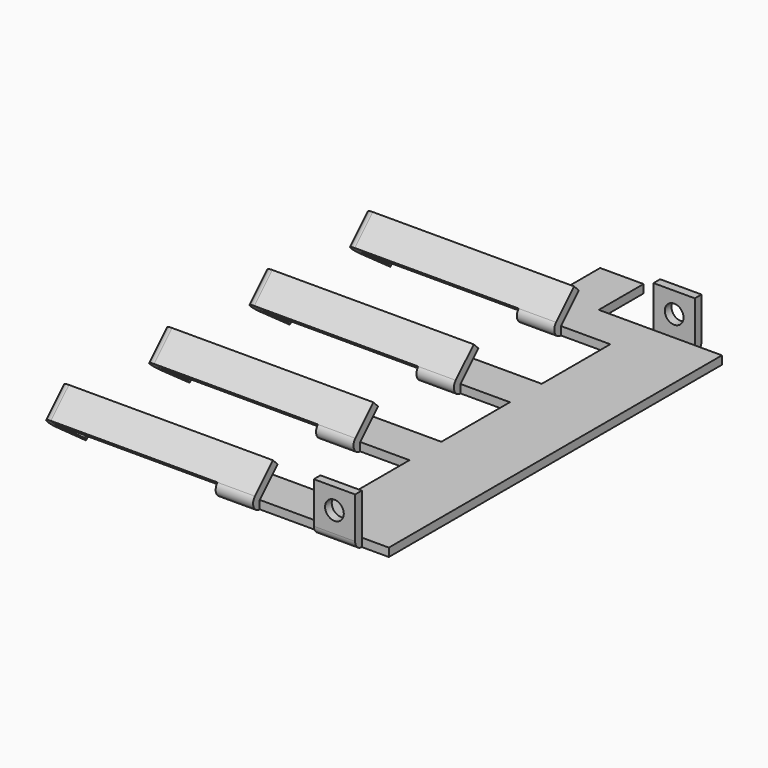
from build123d import *

# Parameters (mm, degrees)
F1_DEPTH  = 1
F3_DEPTH  = 40
F5_DEPTH  = 7.6454254
F8_DEPTH  = 8.9916
F9_DEPTH  = 39.37
F11_REACH = 42.1217729552
F13_REACH = 63.4368099505
F15_REACH = 84.7531019793
F16_W     = 9.9314
F16_H     = 11.938
F17_DEPTH = 2
F18_W     = 9.9314
F18_H     = 11.938
F19_DEPTH = 2
F20_R     = 2
F22_D     = 4.5


with BuildPart() as f1:
    # F0 (on Top) → F1 (new body, symmetric)
    with BuildSketch(Plane.XY):
        Polygon((40, -50), (40, 50), (10.4203875556, 50), (10.4203875556, 63.4358227253), (0, 63.4358227253), (0, 50), (0, 40.4320432043), (20.8407751113, 40.4320432043), (20.8407751113, 19.8559855986), (0, 19.8559855986), (0, 10.2880288029), (20.8407751113, 10.2880288029), (20.8407751113, -10.2880288029), (0, -10.2880288029), (0, -19.8559855986), (20.8407751113, -19.8559855986), (20.8407751113, -40.4320432043), (0, -40.4320432043), (0, -50), align=None)
    extrude(amount=F1_DEPTH, both=True)

    # F2 (on Right) → F3 (join)
    with BuildSketch(Plane.YZ):
        Polygon((-50, 1), (-50, 0.9964082731), (-44.6311706177, 6.3652376554), (-46.04538418, 7.7794512178), (-51.4515079706, 2.3733274272), align=None)
    extrude(amount=-F3_DEPTH)

    # F4 (on face) → F5 (join)
    with BuildSketch(Plane(origin=(0, -19.1329664811, -19.1329664811), x_dir=(1, 0, 0), z_dir=(0, 0.7071067812, 0.7071067812))):
        with BuildLine():
            Line((-34.9300994608, -32.0862576741), (-40.6840402867, -34.1805208645))
            ThreePointArc((-40.6840402867, -34.1805208645), (-41.969615506, -36.4072024614), (-40, -38.059906106))
            Line((-40, -38.059906106), (-40, -36.059906106))
            Line((-40, -36.059906106), (-34.2460591741, -33.9656429157))
            Line((-34.2460591741, -33.9656429157), (-34.9300994608, -32.0862576741))
        make_face()
    extrude(amount=-F5_DEPTH)

    # F6 (on Right) + F2 (on Right) + F7 (on Right) → F8 (join)
    with BuildSketch(Plane.YZ):
        Polygon((-19.8559855986, 0.9982251152), (-19.8559855986, 0.9946333883), (-14.4871562162, 6.3634627706), (-15.9013697786, 7.777676333), (-21.3074935692, 2.3715525424), align=None)
        with BuildLine():
            Line((-19.8559855986, -1), (-19.8559855986, 0.9946333883))
            Line((-19.8559855986, 0.9946333883), (-19.8559855986, 0.9982251152))
            Line((-19.8559855986, 0.9982251152), (-21.3074935692, 2.3715525424))
            ThreePointArc((-21.3074935692, 2.3715525424), (-21.6913494545, 0.2080712521), (-19.8559855986, -1))
        make_face()
    with BuildSketch(Plane.YZ):
        Polygon((-50, 1), (-50, 0.9964082731), (-44.6311706177, 6.3652376554), (-46.04538418, 7.7794512178), (-51.4515079706, 2.3733274272), align=None)
        with BuildLine():
            Line((-50, -0.9982251152), (-50, 0.9964082731))
            Line((-50, 0.9964082731), (-50, 1))
            Line((-50, 1), (-51.4515079706, 2.3733274272))
            ThreePointArc((-51.4515079706, 2.3733274272), (-51.8353638559, 0.2098461369), (-50, -0.9982251152))
        make_face()
    with BuildSketch(Plane.YZ):
        Polygon((10.2880288029, 0.9982251152), (10.2880288029, 0.9946333883), (15.6568581852, 6.3634627706), (14.2426446228, 7.777676333), (8.8365208322, 2.3715525424), align=None)
        with BuildLine():
            Line((10.2880288029, -1), (10.2880288029, 0.9946333883))
            Line((10.2880288029, 0.9946333883), (10.2880288029, 0.9982251152))
            Line((10.2880288029, 0.9982251152), (8.8365208322, 2.3715525424))
            ThreePointArc((8.8365208322, 2.3715525424), (8.4526649469, 0.2080712521), (10.2880288029, -1))
        make_face()
        Polygon((40.4320432043, 1), (40.4320432043, 0.9964082731), (45.8008725867, 6.3652376554), (44.3866590243, 7.7794512177), (38.9805352337, 2.3733274272), align=None)
        with BuildLine():
            Line((40.4320432043, -0.9982251152), (40.4320432043, 0.9964082731))
            Line((40.4320432043, 0.9964082731), (40.4320432043, 1))
            Line((40.4320432043, 1), (38.9805352337, 2.3733274272))
            ThreePointArc((38.9805352337, 2.3733274272), (38.5966793484, 0.2098461369), (40.4320432043, -0.9982251152))
        make_face()
    extrude(amount=F8_DEPTH)

    # F6 (on Right) + F7 (on Right) → F9 (join)
    with BuildSketch(Plane.YZ):
        Polygon((-19.8559855986, 0.9982251152), (-19.8559855986, 0.9946333883), (-14.4871562162, 6.3634627706), (-15.9013697786, 7.777676333), (-21.3074935692, 2.3715525424), align=None)
    with BuildSketch(Plane.YZ):
        Polygon((10.2880288029, 0.9982251152), (10.2880288029, 0.9946333883), (15.6568581852, 6.3634627706), (14.2426446228, 7.777676333), (8.8365208322, 2.3715525424), align=None)
        Polygon((40.4320432043, 1), (40.4320432043, 0.9964082731), (45.8008725867, 6.3652376554), (44.3866590243, 7.7794512177), (38.9805352337, 2.3733274272), align=None)
    extrude(amount=-F9_DEPTH)

    f11_end = Plane(origin=(-19.685, -20.5817395839, 1.6848888288), x_dir=(0, -0.7263986223, 0.6872736293), z_dir=(0, -0.6872736293, -0.7263986223))
    # F10 (on face) → F11 (join, up to a plane its end follows)
    with BuildSketch(Plane(origin=(0, -4.0618467228, -4.0618467228), x_dir=(-1, 0, 0), z_dir=(0, 0.7071067812, 0.7071067812))):
        with BuildLine():
            Line((34.3000994608, 10.7699656456), (40.0540402867, 12.8642288359))
            ThreePointArc((40.0540402867, 12.8642288359), (41.339615506, 15.0909104328), (39.37, 16.7436140775))
            Line((39.37, 16.7436140775), (39.37, 14.7436140775))
            Line((39.37, 14.7436140775), (33.6160591741, 12.6493508872))
            Line((33.6160591741, 12.6493508872), (34.3000994608, 10.7699656456))
        make_face()
    f11_long = extrude(amount=-F11_REACH, mode=Mode.PRIVATE)
    add(split(f11_long, bisect_by=f11_end, keep=Keep.BOTTOM, mode=Mode.PRIVATE))

    f13_end = Plane(origin=(-19.685, 9.5622748176, 1.6848888288), x_dir=(0, -0.7263986223, 0.6872736293), z_dir=(0, -0.6872736293, -0.7263986223))
    # F12 (on face) → F13 (join, up to a plane its end follows)
    with BuildSketch(Plane(origin=(0, 11.0101604779, 11.0101604779), x_dir=(1, 0, 0), z_dir=(0, 0.7071067812, 0.7071067812))):
        with BuildLine():
            Line((-34.3000994608, 10.5450713499), (-40.0540402867, 8.4508081595))
            ThreePointArc((-40.0540402867, 8.4508081595), (-41.339615506, 6.2241265626), (-39.37, 4.5714229179))
            Line((-39.37, 4.5714229179), (-39.37, 6.5714229179))
            Line((-39.37, 6.5714229179), (-33.6160591741, 8.6656861083))
            Line((-33.6160591741, 8.6656861083), (-34.3000994608, 10.5450713499))
        make_face()
    f13_long = extrude(amount=-F13_REACH, mode=Mode.PRIVATE)
    add(split(f13_long, bisect_by=f13_end, keep=Keep.BOTTOM, mode=Mode.PRIVATE))

    f15_end = Plane(origin=(-19.685, 39.706289219, 1.6866637136), x_dir=(0, -0.7263986223, 0.6872736293), z_dir=(0, -0.6872736293, -0.7263986223))
    # F14 (on face) → F15 (join, up to a plane its end follows)
    with BuildSketch(Plane(origin=(0, 26.0830551211, 26.083055121), x_dir=(-1, 0, 0), z_dir=(0, 0.7071067812, 0.7071067812))):
        with BuildLine():
            Line((34.3000994608, -31.8588533121), (40.0540402867, -29.7645901218))
            ThreePointArc((40.0540402867, -29.7645901218), (41.339615506, -27.5379085249), (39.37, -25.8852048802))
            Line((39.37, -25.8852048802), (39.37, -27.8852048802))
            Line((39.37, -27.8852048802), (33.6160591741, -29.9794680706))
            Line((33.6160591741, -29.9794680706), (34.3000994608, -31.8588533121))
        make_face()
    f15_long = extrude(amount=-F15_REACH, mode=Mode.PRIVATE)
    add(split(f15_long, bisect_by=f15_end, keep=Keep.BOTTOM, mode=Mode.PRIVATE))

    # F16 (on face) → F17 (join)
    with BuildSketch(Plane(origin=(0, 50, 0), x_dir=(-1, 0, 0), z_dir=(0, 1, 0))):
        with Locations((-28.5319, 4.969)):
            Rectangle(F16_W, F16_H)
    extrude(amount=F17_DEPTH)

    # F18 (on face) → F19 (join)
    with BuildSketch(Plane.XZ.offset(50)):
        with Locations((28.5319, 4.969)):
            Rectangle(F18_W, F18_H)
    extrude(amount=F19_DEPTH)

    # F20
    f20_edges = [f1.edges().sort_by_distance(p)[0] for p in [
        (28.5319, -52, -1),
        (28.5319, 52, -1),
    ]]
    fillet(f20_edges, radius=F20_R)

    # F22 (through all)
    with Locations(Plane.XZ.offset(52)):
        with Locations((28.5319, 5.9723)):
            Hole(F22_D / 2)


solid = f1.part
